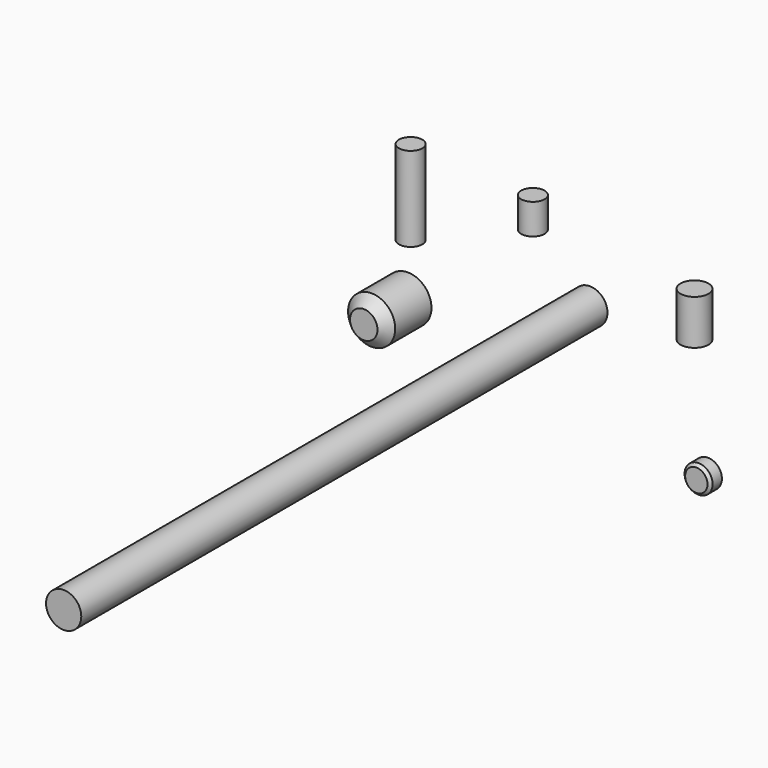
from build123d import *

# Parameters (mm, degrees)
F0_R      = 4.7625
F1_DEPTH  = 177.8
F4_R      = 3.175
F5_DEPTH  = 8.255
F2_R      = 3.175
F6_DEPTH  = 22.86
F8_R      = 3.7846
F9_DEPTH  = 12.13104
F10_R     = 6.3754
F11_DEPTH = 14.90726
F12_SIZE  = 2.667
F13_R     = 3.7846
F14_DEPTH = 3.91668
F15_SIZE  = 0.762


# Not quite as in the source:
# - the program builds the solid bodies; features that only make, move or delete a surface that nothing else refers to are left out


with BuildPart() as f1:
    # F0 (on Front) → F1 (new body)
    with BuildSketch(Plane.XZ):
        Circle(F0_R)
    extrude(amount=F1_DEPTH)


with BuildPart() as f5:
    # F4 (on Top) → F5 (new body)
    with BuildSketch(Plane.XY):
        with Locations((-31.2774516642, 19.8388285935)):
            Circle(F4_R)
    extrude(amount=F5_DEPTH)


with BuildPart() as f6:
    # F2 (on Top) → F6 (new body)
    with BuildSketch(Plane.XY):
        with Locations((-48.4413914382, 0)):
            Circle(F2_R)
    extrude(amount=F6_DEPTH)


with BuildPart() as f9:
    # F8 (on Top) → F9 (new body)
    with BuildSketch(Plane.XY):
        with Locations((26.7817564309, 1.8860386917)):
            Circle(F8_R)
    extrude(amount=F9_DEPTH)


with BuildPart() as f11:
    # F10 (on Front) → F11 (new body)
    with BuildSketch(Plane.XZ):
        with Locations((-49.1946190596, -14.3176335841)):
            Circle(F10_R)
    extrude(amount=F11_DEPTH)

    # F12
    f12_edges = [f11.edges().sort_by_distance(p)[0] for p in [
        (-55.570019, -14.90726, -14.317634),
    ]]
    chamfer(f12_edges, length=F12_SIZE)


with BuildPart() as f14:
    # F13 (on Front) → F14 (new body)
    with BuildSketch(Plane.XZ):
        with Locations((31.9127030671, -29.4398516417)):
            Circle(F13_R)
    extrude(amount=F14_DEPTH)

    # F15
    f15_edges = [f14.edges().sort_by_distance(p)[0] for p in [
        (28.128103, -3.91668, -29.439852),
    ]]
    chamfer(f15_edges, length=F15_SIZE)


solid = Compound([f1.part, f5.part, f6.part, f9.part, f11.part, f14.part])
